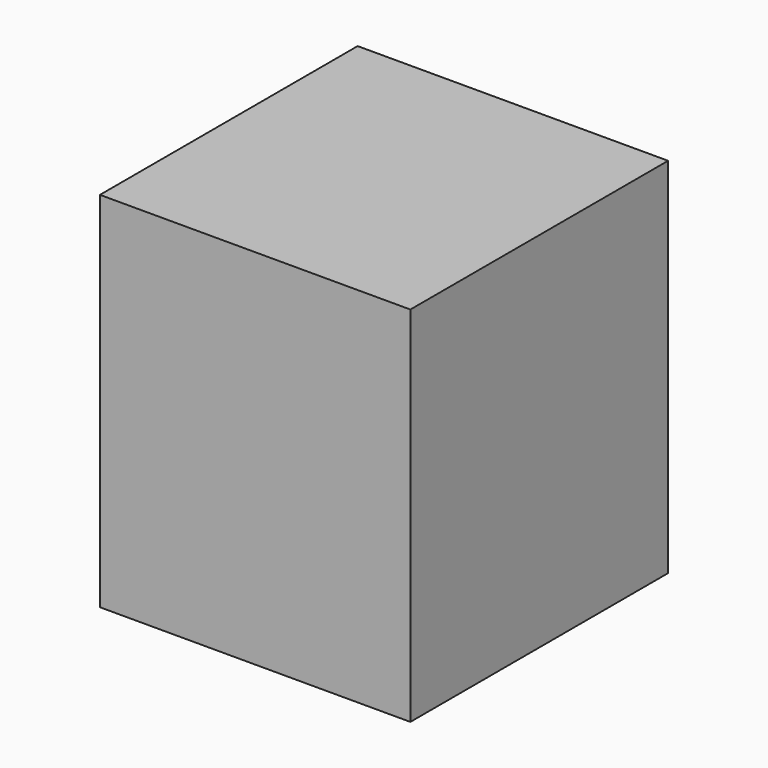
from build123d import *

# Parameters (mm, degrees)
F0_W     = 42.7532605827
F0_H     = 44.3652868271
F1_DEPTH = 50


# Not quite as in the source:
# - the program builds the solid bodies; features that only make, move or delete a surface that nothing else refers to are left out


with BuildPart() as f1:
    # F0 (on Top) → F1 (new body)
    with BuildSketch(Plane.XY):
        with Locations((-5.9790555388, -6.3011422753)):
            Rectangle(F0_W, F0_H)
    extrude(amount=F1_DEPTH)


solid = f1.part
